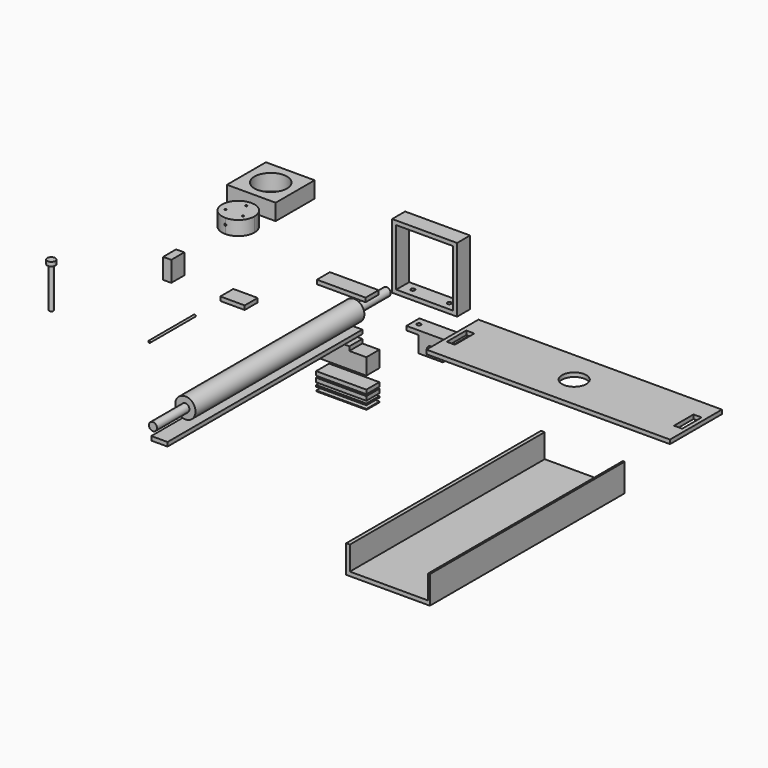
from build123d import *

# Parameters (mm, degrees)
F0_R      = 5
F1_DEPTH  = 20
F0_W      = 60
F0_H      = 5
F0_W_2    = 80
F0_H_2    = 80
F0_W_3    = 70
F0_H_3    = 70
F0_W_4    = 61.861140081
F0_H_4    = 1
F0_H_5    = 2
F0_R_2    = 12.5
F2_DEPTH  = 260
F3_R      = 5
F4_DEPTH  = 50
F5_DEPTH  = 300
F6_R      = 2.5
F7_DEPTH  = 25
F9_R      = 2.5
F8_R      = 2.5
F10_DEPTH = 25
F14_R     = 5
F15_DEPTH = 50
F16_W     = 300
F16_H     = 5
F17_DEPTH = 80
F20_DEPTH = 17.5
F19_W     = 60
F19_H     = 60
F19_R     = 20
F21_DEPTH = 20
F18_W     = 10
F18_H     = 30
F18_R     = 15
F22_DEPTH = 129.4251411048
F18_H_2   = 20
F23_DEPTH = 25
F18_W_2   = 30
F24_DEPTH = 5
F13_R     = 2.5
F25_DEPTH = 5
F26_R     = 5
F27_DEPTH = 5
F28_R     = 2.5
F29_DEPTH = 50
F32_DEPTH = 111.1712381574
F33_R     = 1.25
F34_DEPTH = 70
F35_R     = 1.25
F36_DEPTH = 107.1461310813
F38_DEPTH = 300


# Not quite as in the source:
# - a feature of the source that left no trace in its solid (it failed there, or was rolled back) is left out
# - a feature names something its author has since deleted; it is built from what else it names


with BuildPart() as f1:
    # F0 (on Front) → F1 (new body)
    with BuildSketch(Plane.XZ):
        Polygon((95.2936565876, -7.5), (110.2936565876, -7.5), (125.2936565876, -7.5), (125.2936565876, 12.5), (140.2936565876, 12.5), (140.2936565876, 17.5), (110.2936565876, 17.5), (80.2936565876, 17.5), (80.2936565876, 12.5), (95.2936565876, 12.5), align=None)
        with Locations((110.2936565876, 0)):
            Circle(F0_R, mode=Mode.SUBTRACT)
    extrude(amount=F1_DEPTH)

    # F9 (on face) + F8 (on face) → F10 (cut)
    with BuildSketch(Plane(origin=(0, 0, 12.5), x_dir=(1, 0, 0), z_dir=(0, 0, -1))):
        with Locations((87.7936565876, 10)):
            Circle(F9_R)
    with BuildSketch(Plane(origin=(0, 0, 12.5), x_dir=(1, 0, 0), z_dir=(0, 0, -1))):
        with Locations((132.7936565876, 10)):
            Circle(F8_R)
    extrude(amount=-F10_DEPTH, mode=Mode.SUBTRACT)


with BuildPart() as f1b:
    # F0 (on Front) → F1, piece 2 (new body)
    with BuildSketch(Plane.XZ):
        with Locations((0, 29.2427036911)):
            Rectangle(F0_W, F0_H)
    extrude(amount=F1_DEPTH)


with BuildPart() as f1c:
    # F0 (on Front) → F1, piece 3 (new body)
    with BuildSketch(Plane.XZ):
        Polygon((10, -27.5771580637), (0, -27.5771580637), (-10, -27.5771580637), (-10, -32.5771580637), (-10.9305700405, -32.5771580637), (-30.9305700405, -32.5771580637), (-30.9305700405, -52.5771580637), (0, -52.5771580637), (30.9305700405, -52.5771580637), (30.9305700405, -32.5771580637), (10.9305700405, -32.5771580637), (10, -32.5771580637), align=None)
    extrude(amount=F1_DEPTH)

    # F6 (on face) → F7 (cut)
    with BuildSketch(Plane.XY.offset(-32.5771580637)):
        with Locations((-20, -10)):
            Circle(F6_R)
    extrude(amount=-F7_DEPTH, mode=Mode.SUBTRACT)


with BuildPart() as f1d:
    # F0 (on Front) → F1, piece 4 (new body)
    with BuildSketch(Plane.XZ):
        with Locations((102.7326732874, 87.7068325877)):
            Rectangle(F0_W_2, F0_H_2)
        with Locations((102.7326732874, 87.7068325877)):
            Rectangle(F0_W_3, F0_H_3, mode=Mode.SUBTRACT)
    extrude(amount=F1_DEPTH)

    # F13 (on face) → F25 (cut, through all)
    with BuildSketch(Plane(origin=(0, 0, 47.7068325877), x_dir=(1, 0, 0), z_dir=(0, 0, -1))):
        with Locations((125.2326732874, 10)):
            Circle(F13_R)
        with Locations((80.2326732874, 10)):
            Circle(F13_R)
    extrude(amount=-F25_DEPTH, mode=Mode.SUBTRACT)


with BuildPart() as f1e:
    # F0 (on Front) → F1, piece 5 (new body)
    with BuildSketch(Plane.XZ):
        with Locations((0, -77.355325222)):
            Rectangle(F0_W_4, F0_H)
    extrude(amount=F1_DEPTH)


with BuildPart() as f1f:
    # F0 (on Front) → F1, piece 6 (new body)
    with BuildSketch(Plane.XZ):
        with Locations((0.1928325291, -89.1451310813)):
            Rectangle(F0_W_4, F0_H_4)
    extrude(amount=F1_DEPTH)


with BuildPart() as f1g:
    # F0 (on Front) → F1, piece 7 (new body)
    with BuildSketch(Plane.XZ):
        with Locations((0, -83.756296128)):
            Rectangle(F0_W_4, F0_H_5)
    extrude(amount=F1_DEPTH)


with BuildPart() as f1h:
    # F0 (on Front) → F1, piece 8 (new body)
    with BuildSketch(Plane.XZ):
        with Locations((0, -70.2389810979)):
            Rectangle(F0_W_4, F0_H)
    extrude(amount=F1_DEPTH)


with BuildPart() as f2:
    # F0 (on Front) → F2 (new body)
    with BuildSketch(Plane.XZ):
        Circle(F0_R_2)
    extrude(amount=F2_DEPTH)

    # F3 (on face) → F4 (join)
    with BuildSketch(Plane.XZ.offset(260)):
        Circle(F3_R)
    extrude(amount=F4_DEPTH)

    # F14 (on face) → F15 (join)
    with BuildSketch(Plane(origin=(0, 0, 0), x_dir=(-1, 0, 0), z_dir=(0, 1, 0))):
        Circle(F14_R)
    extrude(amount=F15_DEPTH)


with BuildPart() as f5:
    # F0 (on Front) → F5 (new body)
    with BuildSketch(Plane.XZ):
        Polygon((-10, -22.5167013705), (0, -22.5167013705), (10, -22.5167013705), (10, -17.5167013705), (0, -17.5167013705), (-10, -17.5167013705), align=None)
    extrude(amount=F5_DEPTH)


with BuildPart() as f17:
    # F16 (on Front) → F17 (new body)
    with BuildSketch(Plane.XZ):
        with Locations((303.0256081372, 37.2790100235)):
            Rectangle(F16_W, F16_H)
    extrude(amount=F17_DEPTH)

    # F18 (on face) → F22 (cut, through all)
    with BuildSketch(Plane.XY.offset(39.7790100235)):
        with Locations((163.0256081372, -40)):
            Rectangle(F18_W, F18_H)
        with Locations((443.0256081372, -40)):
            Rectangle(F18_W, F18_H)
        with Locations((303.0256081372, -40)):
            Circle(F18_R)
    extrude(amount=-F22_DEPTH, mode=Mode.SUBTRACT)


with BuildPart() as f20:
    # F19 (on Top) → F20 (new body)
    with BuildSketch(Plane.XY):
        with BuildLine():
            ThreePointArc((-196.265943614, 46.8016631402), (-182.1238079903, 52.6595275165), (-176.265943614, 66.8016631402))
            ThreePointArc((-176.265943614, 66.8016631402), (-210.4080792377, 80.9437987639), (-196.265943614, 46.8016631402))
        make_face()
    extrude(amount=F20_DEPTH)

    # F31 (on face) → F32 (cut, through all)
    with BuildSketch(Plane(origin=(0, 46.8016631402, 0), x_dir=(-1, 0, 0), z_dir=(0, 1, 0))):
        with BuildLine():
            Line((196.265943614, 8.75), (196.265943614, 11.25))
            ThreePointArc((196.265943614, 11.25), (195.015943614, 10), (196.265943614, 8.75))
        make_face()
        with BuildLine():
            ThreePointArc((196.265943614, 8.75), (197.1498270905, 9.1161165235), (197.515943614, 10))
            ThreePointArc((197.515943614, 10), (197.1498270905, 10.8838834765), (196.265943614, 11.25))
            Line((196.265943614, 11.25), (196.265943614, 8.75))
        make_face()
    extrude(amount=F32_DEPTH, mode=Mode.SUBTRACT)

    # F35 (on face) → F36 (cut, through all)
    with BuildSketch(Plane.XY.offset(17.5)):
        with Locations((-196.265943614, 79.3016631402)):
            Circle(F35_R)
        with Locations((-185.4406260667, 60.5516631402)):
            Circle(F35_R)
        with Locations((-207.0912611613, 60.5516631402)):
            Circle(F35_R)
    extrude(amount=-F36_DEPTH, mode=Mode.SUBTRACT)


with BuildPart() as f21:
    # F19 (on Top) → F21 (new body)
    with BuildSketch(Plane.XY):
        with Locations((-205.1943850517, 127.9719012976)):
            Rectangle(F19_W, F19_H)
        with Locations((-205.1943850517, 127.9719012976)):
            Circle(F19_R, mode=Mode.SUBTRACT)
    extrude(amount=F21_DEPTH)


with BuildPart() as f23:
    # F18 (on face) → F23 (new body)
    with BuildSketch(Plane.XY.offset(39.7790100235)):
        with Locations((-130.5344802141, -114.8494374752)):
            Rectangle(F18_W, F18_H_2)
    extrude(amount=F23_DEPTH)


with BuildPart() as f24:
    # F18 (on face) → F24 (new body)
    with BuildSketch(Plane.XY.offset(39.7790100235)):
        with Locations((-50.0688782334, -114.8494374752)):
            Rectangle(F18_W_2, F18_H_2)
    extrude(amount=F24_DEPTH)


with BuildPart() as f27:
    # F26 (on Top) → F27 (new body)
    with BuildSketch(Plane.XY):
        with Locations((-287.8777384163, -106.7102653366)):
            Circle(F26_R)
    extrude(amount=F27_DEPTH)

    # F28 (on face) → F29 (join)
    with BuildSketch(Plane.XY):
        with Locations((-287.7346277237, -106.8533882499)):
            Circle(F28_R)
    extrude(amount=-F29_DEPTH)


with BuildPart() as f34:
    # F33 (on Front) → F34 (new body)
    with BuildSketch(Plane.XZ):
        with Locations((-196.4730769396, -69.498129189)):
            Circle(F33_R)
    extrude(amount=F34_DEPTH)


with BuildPart() as f38:
    # F37 (on Front) → F38 (new body)
    with BuildSketch(Plane.XZ):
        Polygon((330.9895550274, -85.0149002401), (234.6586690965, -85.0149002401), (234.6586690965, -55.713441995), (230.1440447826, -55.713441995), (230.1440447826, -85.0149002401), (230.1440447826, -90.0149002401), (333.2209825259, -90.0149002401), (333.2209825259, -85.0149002401), (333.2209825259, -55.713441995), (330.9895550274, -55.713441995), align=None)
    extrude(amount=F38_DEPTH)


solid = Compound([f1.part, f1b.part, f1c.part, f1d.part, f1e.part, f1f.part, f1g.part, f1h.part, f2.part, f5.part, f17.part, f20.part, f21.part, f23.part, f24.part, f27.part, f34.part, f38.part])
